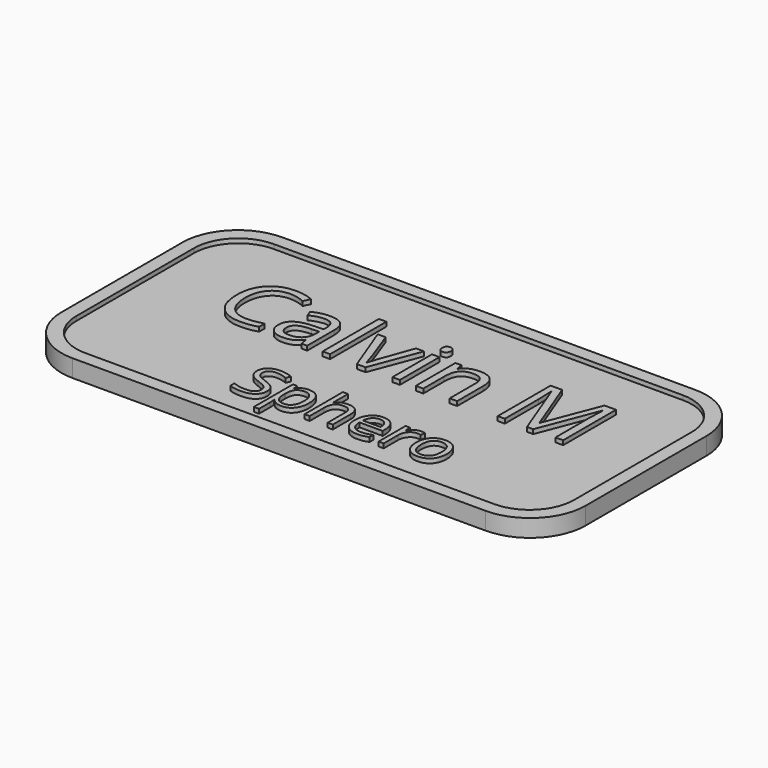
from build123d import *

# Parameters (mm, degrees)
F1_DEPTH       = 1.5
F3_DEPTH       = 0.5
F4_TEXT_SIZE   = 10.5940665688
F4_TEXT_SIZE_2 = 7.2129833926
F5_DEPTH       = 0.5


# Not quite as in the source:
# - Text() gives the source's letters only with a copy of the font that has no kerning and outlines rounded to 1/6400 em; it was checked with that copy


with BuildPart() as f1:
    # F0 (on Top) → F1 (new body)
    with BuildSketch(Plane.XY):
        with BuildLine():
            ThreePointArc((30, 8.65), (28.1401280605, 13.1401280605), (23.65, 15))
            Line((23.65, 15), (-23.65, 15))
            ThreePointArc((-23.65, 15), (-28.1401280605, 13.1401280605), (-30, 8.65))
            Line((-30, 8.65), (-30, -8.65))
            ThreePointArc((-30, -8.65), (-28.1401280605, -13.1401280605), (-23.65, -15))
            Line((-23.65, -15), (23.65, -15))
            ThreePointArc((23.65, -15), (28.1401280605, -13.1401280605), (30, -8.65))
            Line((30, -8.65), (30, 8.65))
        make_face()
    extrude(amount=F1_DEPTH)

    # F2 (on face) → F3 (join)
    with BuildSketch(Plane.XY.offset(1.5)):
        with BuildLine():
            Line((30, -8.65), (30, 8.65))
            ThreePointArc((30, 8.65), (28.1401280605, 13.1401280605), (23.65, 15))
            Line((23.65, 15), (-23.65, 15))
            ThreePointArc((-23.65, 15), (-28.1401280605, 13.1401280605), (-30, 8.65))
            Line((-30, 8.65), (-30, -8.65))
            ThreePointArc((-30, -8.65), (-28.1401280605, -13.1401280605), (-23.65, -15))
            Line((-23.65, -15), (23.65, -15))
            ThreePointArc((23.65, -15), (28.1401280605, -13.1401280605), (30, -8.65))
        make_face()
        with BuildLine():
            Line((-23.42, 13.5), (23.42, 13.5))
            ThreePointArc((23.42, 13.5), (27.0121024484, 12.0121024484), (28.5, 8.42))
            Line((28.5, 8.42), (28.5, -8.42))
            ThreePointArc((28.5, -8.42), (27.0121024484, -12.0121024484), (23.42, -13.5))
            Line((23.42, -13.5), (-23.42, -13.5))
            ThreePointArc((-23.42, -13.5), (-27.0121024484, -12.0121024484), (-28.5, -8.42))
            Line((-28.5, -8.42), (-28.5, 8.42))
            ThreePointArc((-28.5, 8.42), (-27.0121024484, 12.0121024484), (-23.42, 13.5))
        make_face(mode=Mode.SUBTRACT)
    extrude(amount=F3_DEPTH)

    # F4 (on face) → F5 (join)
    with BuildSketch(Plane.XY.offset(1.5)):
        with Locations((-20.5135890552, 0)):
            Text('Calvin M', F4_TEXT_SIZE, font='Open Sans', text_align=(TextAlign.LEFT, TextAlign.BOTTOM))
        with Locations((-9.6933357418, -10.4979379103)):
            Text('Sphero', F4_TEXT_SIZE_2, font='Open Sans', text_align=(TextAlign.LEFT, TextAlign.BOTTOM))
    extrude(amount=F5_DEPTH)


solid = f1.part
